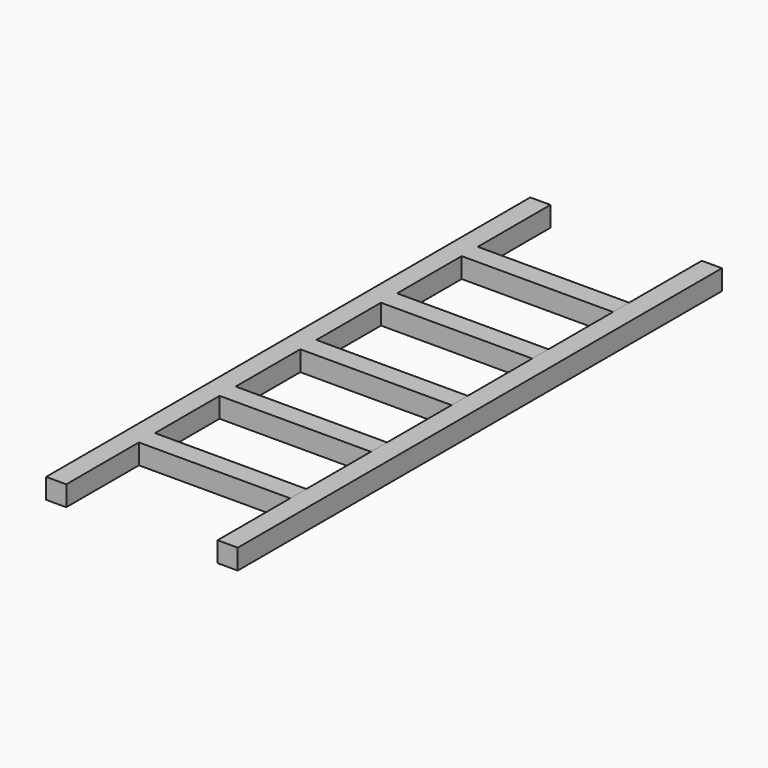
from build123d import *

# Parameters (mm, degrees)
F0_W     = 2
F0_H     = 2
F1_DEPTH = 60
F2_W     = 2
F2_H     = 2
F3_DEPTH = 15


with BuildPart() as f1:
    # F0 (on Front) → F1 (new body)
    with BuildSketch(Plane.XZ):
        with Locations((-29.2174071148, 15.274727294)):
            Rectangle(F0_W, F0_H)
    extrude(amount=F1_DEPTH)

    # F2 (on face) → F3 (join)
    with BuildSketch(Plane.YZ.offset(-28.2174071148)):
        with Locations((-50, 15.274727294)):
            Rectangle(F2_W, F2_H)
        with Locations((-40, 15.274727294)):
            Rectangle(F2_W, F2_H)
        with Locations((-30, 15.274727294)):
            Rectangle(F2_W, F2_H)
        with Locations((-20, 15.274727294)):
            Rectangle(F2_W, F2_H)
        with Locations((-10, 15.274727294)):
            Rectangle(F2_W, F2_H)
    extrude(amount=F3_DEPTH)


with BuildPart() as f1b:
    # F0 (on Front) → F1, piece 2 (new body)
    with BuildSketch(Plane.XZ):
        with Locations((-12.2174071148, 15.274727294)):
            Rectangle(F0_W, F0_H)
    extrude(amount=F1_DEPTH)


solid = Compound([f1.part, f1b.part])
